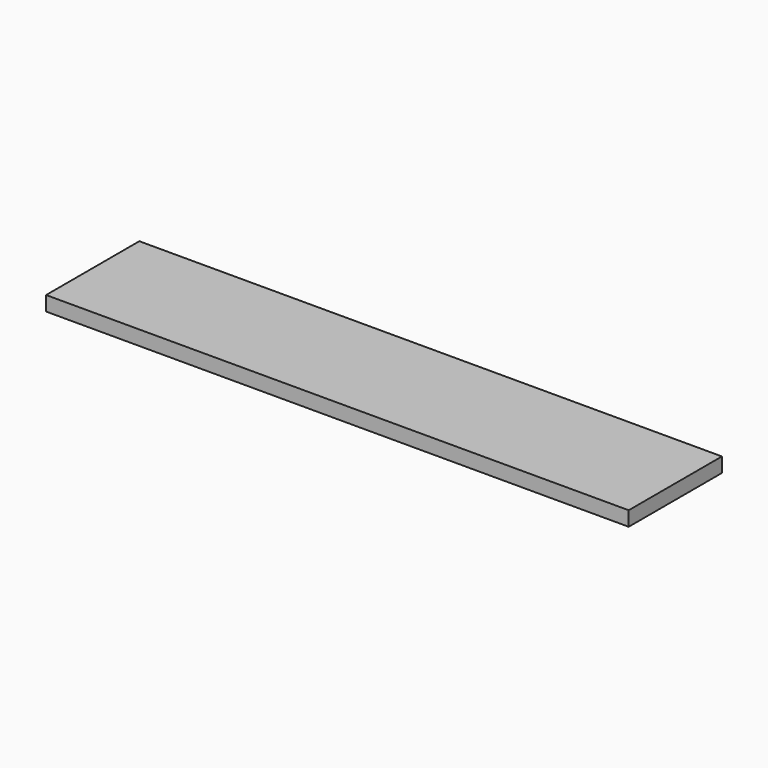
from build123d import *

# Parameters (mm, degrees)
F0_W     = 381
F0_H     = 76.2
F1_DEPTH = 9.525


# Not quite as in the source:
# - a length typed as a fraction of an inch, garbled in the dataset ("3 / 203.2 mm" for 3/8 in), is restored


with BuildPart() as f1:
    # F0 (on Top) → F1 (new body)
    with BuildSketch(Plane.XY):
        Rectangle(F0_W, F0_H)
    extrude(amount=F1_DEPTH)


solid = f1.part
